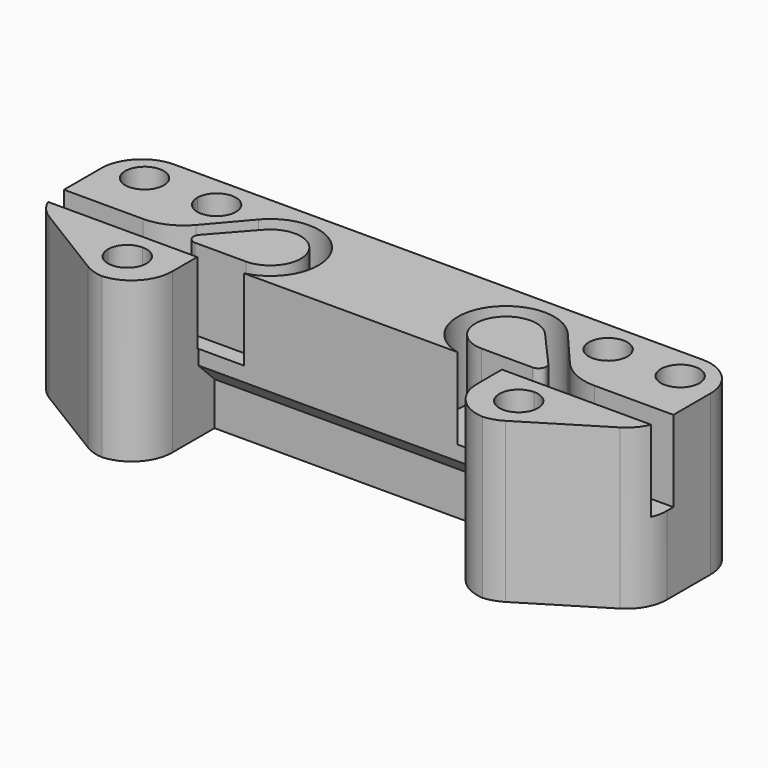
from build123d import *

# Parameters (mm, degrees)
F1_DEPTH    = 15.7
F2_W        = 10.0960650777
F2_H        = 2.35
F3_DEPTH    = 8
F4_R        = 5
F5_T1_DEPTH = 26.8923143391
F5_T3_DEPTH = 21.3473434867
F5_T5_DEPTH = 35.7
F6_W        = 15
F6_H        = 6.25
F7_DEPTH    = 2
F8_SIZE     = 1.99999


# Not quite as in the source:
# - a fillet or chamfer that OpenCascade refuses, or shapes differently, is made with other operations: its cross-section is extruded or revolved along the edge and cut away or added
# - a fillet or chamfer is up to 0.001 mm smaller than in the source, because OpenCascade refuses the exact size


with BuildPart() as f1:
    # F0 (on Top) → F1 (new body)
    with BuildSketch(Plane.XY):
        Polygon((30, 9), (0, 9), (0, -1.8), (15, -1.8), (15, -9), (19.5954625243, -9), (30, -2.6151265483), align=None)
        with BuildLine():
            ThreePointArc((21.17, -5.2), (17.9264971157, -6.5435028843), (19.27, -3.3))
            ThreePointArc((19.27, -3.3), (20.6135028843, -3.8564971157), (21.17, -5.2))
        make_face(mode=Mode.SUBTRACT)
        with BuildLine():
            ThreePointArc((19.27, 3.9), (17.9264971157, 7.1435028843), (21.17, 5.8))
            ThreePointArc((21.17, 5.8), (20.6135028843, 4.4564971157), (19.27, 3.9))
        make_face(mode=Mode.SUBTRACT)
        with BuildLine():
            ThreePointArc((24.47, 5.8), (26.37, 7.7), (28.27, 5.8))
            ThreePointArc((28.27, 5.8), (26.37, 3.9), (24.47, 5.8))
        make_face(mode=Mode.SUBTRACT)
    extrude(amount=F1_DEPTH)

    # F2 (on face) → F3 (cut)
    with BuildSketch(Plane.XY.offset(15.7)):
        with BuildLine():
            ThreePointArc((11.6039349223, -0.1749693412), (8.8681704068, 4.0561246908), (13.8492571677, 4.8146356484))
            Line((13.8492571677, 4.8146356484), (16.291649806, 2.0583304766))
            ThreePointArc((16.291649806, 2.0583304766), (16.3383380366, 2.4404176698), (16.3539349223, 2.8250306588))
            ThreePointArc((16.3539349223, 2.8250306588), (16.0600367861, 4.4699185515), (15.2147112678, 5.9112571869))
            ThreePointArc((15.2147112678, 5.9112571869), (7.5463441808, 5.2945361506), (10.5215341623, -1.8))
            Line((10.5215341623, -1.8), (12.6863356823, -1.8))
            ThreePointArc((12.6863356823, -1.8), (14.1212348386, -1.2030831841), (15.286664888, -0.1749693412))
            Line((15.286664888, -0.1749693412), (11.6039349223, -0.1749693412))
        make_face()
        with BuildLine():
            ThreePointArc((16.3539349223, 2.8250306588), (16.3383380366, 2.4404176698), (16.291649806, 2.0583304766))
            Line((16.291649806, 2.0583304766), (17.1652654837, 1.0724319062))
            ThreePointArc((17.1652654837, 1.0724319062), (17.3051830671, 0.8410213344), (17.3539349223, 0.5750306588))
            ThreePointArc((17.3539349223, 0.5750306588), (17.1342650082, 0.0447005729), (16.6039349223, -0.1749693412))
            Line((16.6039349223, -0.1749693412), (15.286664888, -0.1749693412))
            ThreePointArc((15.286664888, -0.1749693412), (14.1212348386, -1.2030831841), (12.6863356823, -1.8))
            Line((12.6863356823, -1.8), (15, -1.8))
            Line((15, -1.8), (15, -1.9249693412))
            Line((15, -1.9249693412), (19.9039349223, -1.9249693412))
            Line((19.9039349223, -1.9249693412), (19.9039349223, 0.4250306588))
            Line((19.9039349223, 0.4250306588), (15.2147112678, 5.9112571869))
            ThreePointArc((15.2147112678, 5.9112571869), (16.0600367861, 4.4699185515), (16.3539349223, 2.8250306588))
        make_face()
        with Locations((24.9519674612, -0.7499693412)):
            Rectangle(F2_W, F2_H)
    extrude(amount=-F3_DEPTH, mode=Mode.SUBTRACT)

    # F4
    f4_edges = [f1.edges().sort_by_distance(p)[0] for p in [
        (19.903935, 0.425031, 11.7),
    ]]
    fillet(f4_edges, radius=F4_R)

    # F5: fillet of radius 4 on 4 edges, made by hand

    # F5_s2 → F5_t1 (cut)
    with BuildSketch(Plane.XY.offset(-5.5961571696)):
        with BuildLine():
            ThreePointArc((30, -0.3766636805), (29.4905957559, -2.3300559271), (28.0921293656, -3.7859150232))
            Line((28.0921293656, -3.7859150232), (30, -2.6151265483))
            Line((30, -2.6151265483), (30, -0.3766636805))
        make_face()
    extrude(amount=F5_T1_DEPTH, mode=Mode.SUBTRACT)

    # F5_s4 → F5_t3 (cut)
    with BuildSketch(Plane.XY.offset(-2.8236717433)):
        with BuildLine():
            ThreePointArc((20.5581231925, -8.4092513427), (19.5529608525, -8.8494808332), (18.465993827, -9))
            Line((18.465993827, -9), (19.5954625243, -9))
            Line((19.5954625243, -9), (20.5581231925, -8.4092513427))
        make_face()
    extrude(amount=F5_T3_DEPTH, mode=Mode.SUBTRACT)

    # F5_s6 → F5_t5 (cut)
    with BuildSketch(Plane.XY.offset(-10)):
        with BuildLine():
            ThreePointArc((15, -5), (16.1715728753, -7.8284271247), (19, -9))
            Line((19, -9), (15, -9))
            Line((15, -9), (15, -5))
        make_face()
        with BuildLine():
            ThreePointArc((30, 5), (28.8284271247, 7.8284271247), (26, 9))
            Line((26, 9), (30, 9))
            Line((30, 9), (30, 5))
        make_face()
    extrude(amount=F5_T5_DEPTH, mode=Mode.SUBTRACT)

    # F6 (on face) → F7 (cut)
    with BuildSketch(Plane.XZ.offset(1.8)):
        with Locations((7.5, 3.125)):
            Rectangle(F6_W, F6_H)
    extrude(amount=-F7_DEPTH, mode=Mode.SUBTRACT)

    # F8 (size 2 in the source; OpenCascade refuses exactly that, so slightly less here)
    f8_edges = [f1.edges().sort_by_distance(p)[0] for p in [
        (7.5, 0.2, 6.25),
    ]]
    chamfer(f8_edges, length=F8_SIZE)

    # F9: F1 across plane


with BuildPart() as f1_1:
    add(f1.part)
    add(f1.part.mirror(Plane.YZ))


solid = f1_1.part
